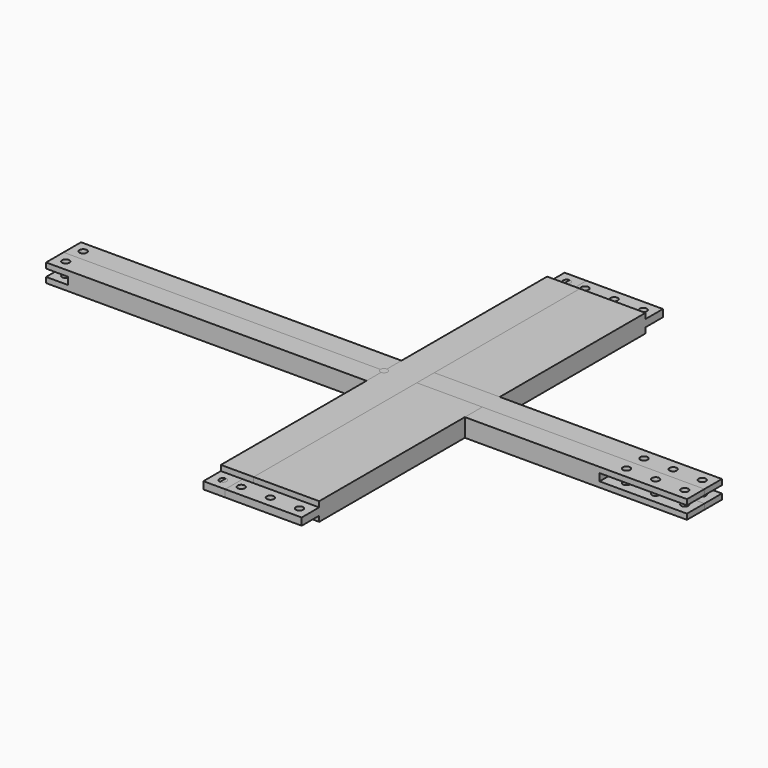
from build123d import *

# Parameters (mm, degrees)
F1_DEPTH  = 19.05
F2_W      = 9.525
F2_H      = 6.35
F3_DEPTH  = 539.751
F4_R      = 3.175
F5_DEPTH  = 15.876
F7_DEPTH  = 85.725
F8_R      = 3.175
F9_DEPTH  = 11.1135
F10_W     = 9.525
F10_H     = 6.35
F11_DEPTH = 393.701
F14_DEPTH = 28.575
F15_W     = 9.525
F15_H     = 6.35
F16_DEPTH = 393.701
F17_R     = 3.175
F18_DEPTH = 11.1135
F19_R     = 3.175
F20_DEPTH = 15.875


with BuildPart() as f1:
    # F0 (on Front) → F1 (new body)
    with BuildSketch(Plane.XZ):
        Polygon((-279.4, 0), (0, 0), (279.4, 0), (279.4, 4.7625), (203.2, 4.7625), (203.2, 11.1125), (279.4, 11.1125), (279.4, 15.875), (0, 15.875), (-279.4, 15.875), (-279.4, 11.1125), (-260.35, 11.1125), (-260.35, 4.7625), (-279.4, 4.7625), align=None)
    extrude(amount=F1_DEPTH)

    # F2 (on face) → F3 (cut, through all)
    with BuildSketch(Plane(origin=(-260.35, 0, 0), x_dir=(0, -1, 0), z_dir=(-1, 0, 0))):
        with Locations((4.7625, 7.9375)):
            Rectangle(F2_W, F2_H)
    extrude(amount=-F3_DEPTH, mode=Mode.SUBTRACT)

    # F4 (on face) → F5 (cut, through all)
    with BuildSketch(Plane.XY.offset(15.875)):
        with Locations((-269.875, -9.525)):
            Circle(F4_R)
        with Locations((269.875, -9.525)):
            Circle(F4_R)
        with Locations((244.475, -9.525)):
            Circle(F4_R)
        with Locations((219.075, -9.525)):
            Circle(F4_R)
    extrude(amount=-F5_DEPTH, mode=Mode.SUBTRACT)


with BuildPart() as f7:
    # F6 (on Right) → F7 (new body)
    with BuildSketch(Plane.YZ):
        Polygon((-177.8, 0), (0, 0), (177.8, 0), (177.8, 4.7625), (196.85, 4.7625), (196.85, 11.1125), (177.8, 11.1125), (177.8, 15.875), (0, 15.875), (-177.8, 15.875), (-177.8, 11.1125), (-196.85, 11.1125), (-196.85, 4.7625), (-177.8, 4.7625), align=None)
    extrude(amount=F7_DEPTH)

    # F8 (on face) → F9 (cut, through all)
    with BuildSketch(Plane.XY.offset(11.1125)):
        with Locations((76.2, 187.325)):
            Circle(F8_R)
        with Locations((76.2, -187.325)):
            Circle(F8_R)
        with Locations((50.8, 187.325)):
            Circle(F8_R)
        with Locations((50.8, -187.325)):
            Circle(F8_R)
        with Locations((25.4, 187.325)):
            Circle(F8_R)
        with Locations((25.4, -187.325)):
            Circle(F8_R)
    extrude(amount=-F9_DEPTH, mode=Mode.SUBTRACT)

    # F10 (on face) → F11 (cut, through all)
    with BuildSketch(Plane.XZ.offset(196.85)):
        with Locations((4.7625, 7.9375)):
            Rectangle(F10_W, F10_H)
    extrude(amount=-F11_DEPTH, mode=Mode.SUBTRACT)


with BuildPart() as f12_1:
    # F12: instance of F1
    add(f1.part.mirror(Plane.XZ))


with BuildPart() as f14:
    # F13 (on Right) → F14 (new body)
    with BuildSketch(Plane.YZ):
        Polygon((-177.8, 0), (0, 0), (177.8, 0), (177.8, 4.7625), (196.85, 4.7625), (196.85, 11.1125), (177.8, 11.1125), (177.8, 15.875), (0, 15.875), (-177.8, 15.875), (-177.8, 11.1125), (-196.85, 11.1125), (-196.85, 4.7625), (-177.8, 4.7625), align=None)
    extrude(amount=F14_DEPTH)

    # F15 (on face) → F16 (cut, through all)
    with BuildSketch(Plane.XZ.offset(196.85)):
        with Locations((23.8125, 7.9375)):
            Rectangle(F15_W, F15_H)
    extrude(amount=-F16_DEPTH, mode=Mode.SUBTRACT)

    # F17 (on face) → F18 (cut, through all)
    with BuildSketch(Plane.XY.offset(11.1125)):
        with Locations((9.525, 187.325)):
            Circle(F17_R)
        with Locations((9.525, -187.325)):
            Circle(F17_R)
    extrude(amount=-F18_DEPTH, mode=Mode.SUBTRACT)


with BuildPart() as f20:
    # F19 (on Top) → F20 (new body)
    with BuildSketch(Plane.XY):
        Circle(F19_R)
    extrude(amount=F20_DEPTH)


solid = Compound([f1.part, f7.part, f12_1.part, f14.part, f20.part])
